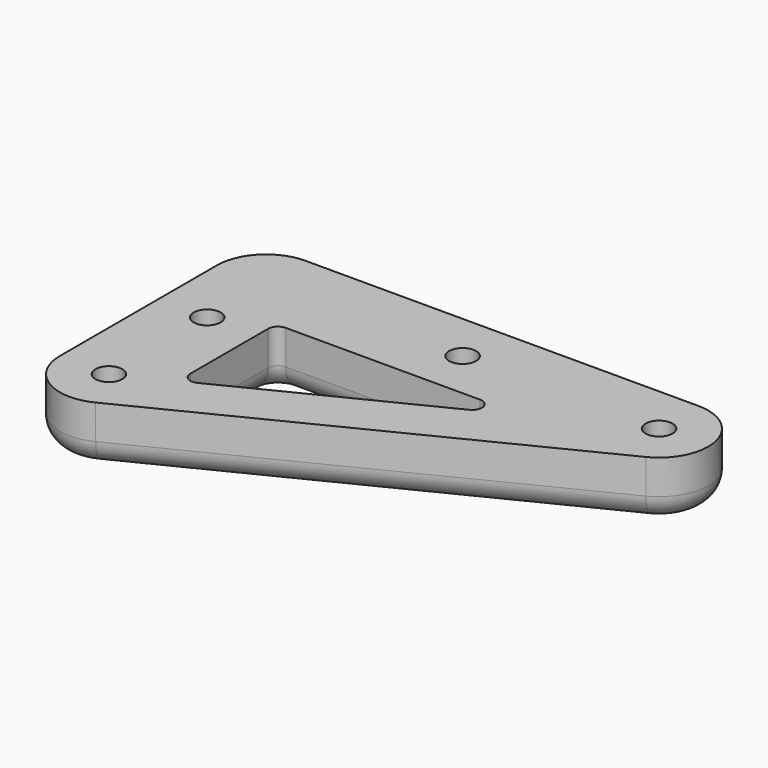
from build123d import *

# Parameters (mm, degrees)
F1_DEPTH       = 12
F2_D           = 5.5
F2_CBORE_D     = 9.75
F2_CBORE_DEPTH = 5
F3_R           = 4.99999


# Not quite as in the source:
# - a fillet or chamfer is up to 0.001 mm smaller than in the source, because OpenCascade refuses the exact size


with BuildPart() as f1:
    # F0 (on Top) → F1 (new body)
    with BuildSketch(Plane.XY):
        with BuildLine():
            Line((80, 10), (0, 10))
            ThreePointArc((0, 10), (-7.0710678119, 7.0710678119), (-10, 0))
            Line((-10, 0), (-10, -40))
            ThreePointArc((-10, -40), (-5.2573111212, -48.5065080835), (4.472135955, -48.94427191))
            Line((4.472135955, -48.94427191), (84.472135955, -8.94427191))
            ThreePointArc((84.472135955, -8.94427191), (89.7324898947, 2.2975292055), (80, 10))
        make_face()
        with BuildLine():
            ThreePointArc((51.527864045, -10), (53.4743620239, -11.5404941589), (52.422291236, -13.788854382))
            Line((52.422291236, -13.788854382), (12.894427191, -33.5527864045))
            ThreePointArc((12.894427191, -33.5527864045), (10.9485377758, -33.4652336392), (10, -31.7639320225))
            Line((10, -31.7639320225), (10, -12))
            ThreePointArc((10, -12), (10.5857864376, -10.5857864376), (12, -10))
            Line((12, -10), (51.527864045, -10))
        make_face(mode=Mode.SUBTRACT)
    extrude(amount=F1_DEPTH)

    # F2 (through all)
    with Locations(Plane(origin=(0, 0, 0), x_dir=(1, 0, 0), z_dir=(0, 0, -1))):
        with Locations((80, 0), (0, 40), (40, 0), (0, 15)):
            CounterBoreHole(F2_D / 2, F2_CBORE_D / 2, F2_CBORE_DEPTH)

    # F3 (radius 5 in the source; OpenCascade refuses exactly that, so slightly less here)
    f3_edges = [f1.edges().sort_by_distance(p)[0] for p in [
        (44.472136, -28.944272, 0),
        (31.763932, -10, 0),
    ]]
    fillet(f3_edges, radius=F3_R)


solid = f1.part
